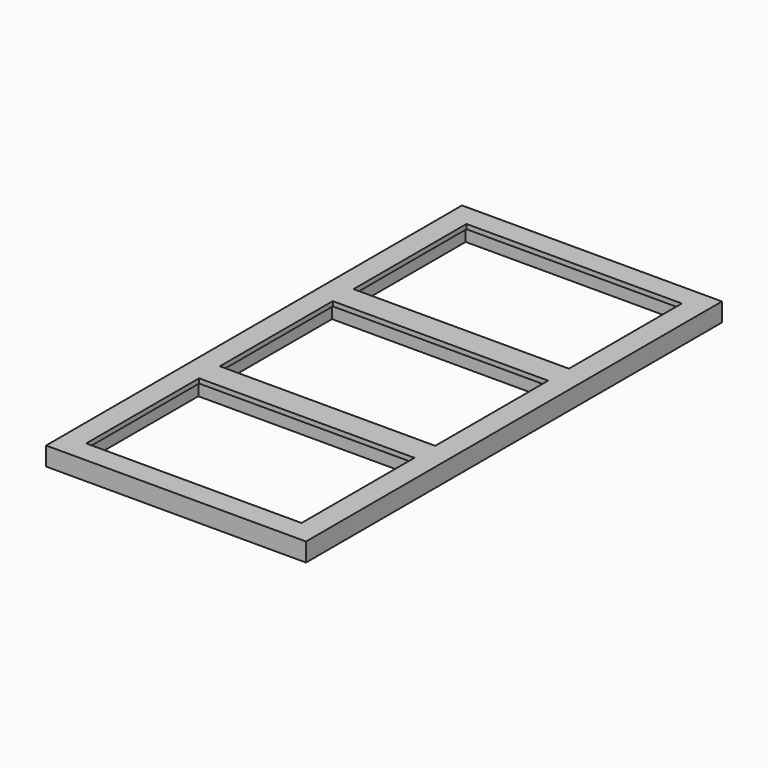
from build123d import *

# Parameters (mm, degrees)
F0_W     = 177.8
F0_H     = 355.6
F2_DEPTH = 12.7
F1_W     = 147.32
F1_H     = 96.52
F4_DEPTH = 12.701
F8_W     = 152.4
F8_H     = 101.6
F9_DEPTH = 9.525


# Not quite as in the source:
# - a length typed as a fraction of an inch, garbled in the dataset ("3 / 203.2 mm" for 3/8 in), is restored


with BuildPart() as f2:
    # F0 (on Top) → F2 (new body)
    with BuildSketch(Plane.XY):
        Rectangle(F0_W, F0_H)
    extrude(amount=-F2_DEPTH)

    # F1 (on face) → F4 (cut, through all)
    with BuildSketch(Plane.XY):
        with Locations((0, -114.3)):
            Rectangle(F1_W, F1_H)
        Rectangle(F1_W, F1_H)
        with Locations((0, 114.3)):
            Rectangle(F1_W, F1_H)
    extrude(amount=-F4_DEPTH, mode=Mode.SUBTRACT)

    # F8 (on face) → F9 (cut)
    with BuildSketch(Plane(origin=(0, 0, -12.7), x_dir=(1, 0, 0), z_dir=(0, 0, -1))):
        with Locations((0, -114.3)):
            Rectangle(F8_W, F8_H)
        Rectangle(F8_W, F8_H)
        with Locations((0, 114.3)):
            Rectangle(F8_W, F8_H)
    extrude(amount=-F9_DEPTH, mode=Mode.SUBTRACT)


solid = f2.part
